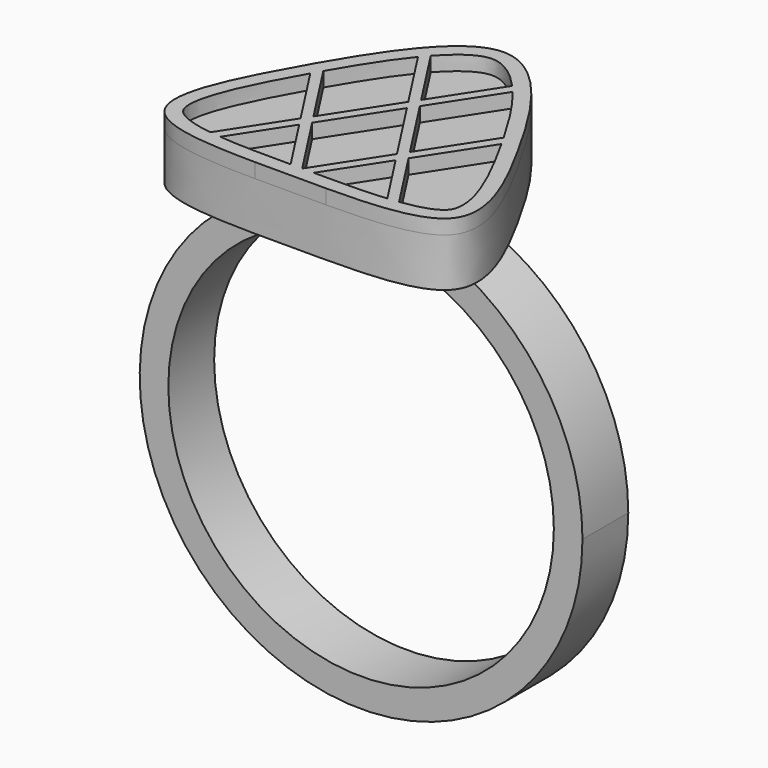
from build123d import *

# Parameters (mm, degrees)
F0_R     = 11.6
F0_R_2   = 10.1
F1_DEPTH = 3
F4_DEPTH = 2.54
F6_DEPTH = 0.762


# Not quite as in the source:
# - ends of sketch curves that miss each other by under 0.0002 mm in the source are joined
# - the dataset's text gives a spline's control points without its knots; the knots are read off the source's solid


with BuildPart() as f1:
    # F0 (on Front) → F1 (new body)
    with BuildSketch(Plane.XZ):
        Circle(F0_R)
        Circle(F0_R_2, mode=Mode.SUBTRACT)
    extrude(amount=F1_DEPTH)

    # F3 (on offset) → F4 (join)
    with BuildSketch(Plane.XY.offset(11.5951)):
        with BuildLine():
            add(Edge.make_bspline(
                [(0, 6.35), (-2.0779078975, 6.35), (-5.972334255, 0.1462705205), (-9.7622210706, -7.761600403), (0, -7.5463996638), (9.7622210706, -7.761600403), (5.972334255, 0.1462705205), (2.0779078975, 6.35), (0, 6.35)],
                knots=[0, 0, 0, 0, 0.1772793323, 0.3322578951, 0.5, 0.6677421049, 0.8227206677, 1, 1, 1, 1], degree=3))
        make_face()
    extrude(amount=F4_DEPTH)

    # F5 (on face) → F6 (join)
    with BuildSketch(Plane.XY.offset(14.1351)):
        with BuildLine():
            add(Edge.make_bspline(
                [(1.8621309249, -7.6179364202), (4.5064725103, -7.597781529), (9.5238408191, -7.2642028945), (5.972334255, 0.1462705205), (2.0779078975, 6.35), (0, 6.35)],
                knots=[0.5314495212, 0.5314495212, 0.5314495212, 0.5314495212, 0.6677421049, 0.8227206677, 1, 1, 1, 1], degree=3))
            add(Edge.make_bspline(
                [(0, 6.35), (-2.0779078975, 6.35), (-5.972334255, 0.1462705205), (-9.5238408191, -7.2642028945), (-4.5064725103, -7.597781529), (-1.8621309249, -7.6179364202)],
                knots=[0, 0, 0, 0, 0.1772793323, 0.3322578951, 0.4685504788, 0.4685504788, 0.4685504788, 0.4685504788], degree=3))
            add(Edge.make_bspline(
                [(-1.8621309249, -7.6179364202), (-1.2480712309, -7.573857345), (0, -7.5189419826), (1.2480712309, -7.573857345), (1.8621309249, -7.6179364202)],
                knots=[0.4788567979, 0.4788567979, 0.4788567979, 0.4788567979, 0.5, 0.5211432021, 0.5211432021, 0.5211432021, 0.5211432021], degree=3))
        make_face()
        with BuildLine():
            add(Edge.make_bspline(
                [(-2.4816082782, 3.8281001657), (-2.5343802796, 3.7637274985), (-2.9162768938, 3.2882987067), (-3.6254819159, 2.2796916192), (-4.3137688684, 1.1448648199), (-4.6726591189, 0.5221257557), (-4.7250085334, 0.4306953674)],
                knots=[0.088736613, 0.088736613, 0.088736613, 0.088736613, 0.09375, 0.125, 0.15625, 0.1616197523, 0.1616197523, 0.1616197523, 0.1616197523], degree=3))
            add(Edge.make_bspline(
                [(-2.1365586498, 4.2296753486), (-2.2511551272, 4.102891236), (-2.366322216, 3.9687291188), (-2.4816082782, 3.8281001657)],
                knots=[0.0777843348, 0.0777843348, 0.0777843348, 0.0777843348, 0.088736613, 0.088736613, 0.088736613, 0.088736613], degree=3))
            add(Edge.make_bspline(
                [(0, 5.588), (-0.0564230571, 5.588), (-0.1692691714, 5.580201891), (-0.4101970388, 5.5316620699), (-0.7423807218, 5.4027827261), (-1.186352477, 5.126577291), (-1.6554698528, 4.7353575108), (-1.9766347616, 4.4066075606), (-2.1365586498, 4.2296753486)],
                knots=[0, 0, 0, 0, 0.0078125, 0.015625, 0.03125, 0.046875, 0.0625, 0.0777843348, 0.0777843348, 0.0777843348, 0.0777843348], degree=3))
            add(Edge.make_bspline(
                [(2.1365586498, 4.2296753486), (1.9766347616, 4.4066075606), (1.6554698528, 4.7353575108), (1.186352477, 5.126577291), (0.7423807218, 5.4027827261), (0.4101970388, 5.5316620699), (0.1692691714, 5.580201891), (0.0564230571, 5.588), (0, 5.588)],
                knots=[0.9222156652, 0.9222156652, 0.9222156652, 0.9222156652, 0.9375, 0.953125, 0.96875, 0.984375, 0.9921875, 1, 1, 1, 1], degree=3))
            add(Edge.make_bspline(
                [(2.4816082782, 3.8281001657), (2.366322216, 3.9687291188), (2.2511551272, 4.102891236), (2.1365586498, 4.2296753486)],
                knots=[0.911263387, 0.911263387, 0.911263387, 0.911263387, 0.9222156652, 0.9222156652, 0.9222156652, 0.9222156652], degree=3))
            add(Edge.make_bspline(
                [(4.7250085334, 0.4306953674), (4.6726591189, 0.5221257557), (4.3137688684, 1.1448648199), (3.6254819159, 2.2796916192), (2.9162768938, 3.2882987067), (2.5343802796, 3.7637274985), (2.4816082782, 3.8281001657)],
                knots=[0.8383802477, 0.8383802477, 0.8383802477, 0.8383802477, 0.84375, 0.875, 0.90625, 0.911263387, 0.911263387, 0.911263387, 0.911263387], degree=3))
            add(Edge.make_bspline(
                [(5.0073229685, -0.0677201042), (4.9141625319, 0.0983598325), (4.8200413076, 0.26471675), (4.7250085334, 0.4306953674)],
                knots=[0.8286322408, 0.8286322408, 0.8286322408, 0.8286322408, 0.8383802477, 0.8383802477, 0.8383802477, 0.8383802477], degree=3))
            add(Edge.make_bspline(
                [(4.9439608161, -6.6925174845), (4.9858176889, -6.6868380172), (5.254154786, -6.6488274862), (5.7121852058, -6.5640205362), (6.2365479646, -6.4129993057), (6.6366004374, -6.2332169395), (6.8546525359, -6.0751763267), (6.9682464356, -5.9541298184), (7.0495464906, -5.8365993116), (7.1250231512, -5.653747574), (7.1675880901, -5.3285920553), (7.1372157684, -4.8940903912), (7.0250329785, -4.3683523575), (6.770198138, -3.5694722363), (6.2740558144, -2.4244183762), (5.6110952095, -1.1558825717), (5.1662615974, -0.351188467), (5.0121706035, -0.0763621301), (5.0073229685, -0.0677201042)],
                knots=[0.5909001737, 0.5909001737, 0.5909001737, 0.5909001737, 0.59375, 0.609375, 0.625, 0.640625, 0.65625, 0.6640625, 0.671875, 0.6875, 0.703125, 0.71875, 0.734375, 0.75, 0.78125, 0.8125, 0.828125, 0.8286322408, 0.8286322408, 0.8286322408, 0.8286322408], degree=3))
            add(Edge.make_bspline(
                [(4.3797296074, -6.7559609058), (4.5755658638, -6.7379434213), (4.7640552636, -6.7169284748), (4.9439608161, -6.6925174845)],
                knots=[0.5786512993, 0.5786512993, 0.5786512993, 0.5786512993, 0.5909001737, 0.5909001737, 0.5909001737, 0.5909001737], degree=3))
            add(Edge.make_bspline(
                [(0.6050961097, -6.8584772032), (0.7141147867, -6.8585902422), (1.1322874105, -6.8589569218), (2.154823412, -6.8572987447), (3.3261548926, -6.8341482776), (4.1215009809, -6.7797186631), (4.3797296074, -6.7559609058)],
                knots=[0.5101325373, 0.5101325373, 0.5101325373, 0.5101325373, 0.515625, 0.53125, 0.5625, 0.5786512993, 0.5786512993, 0.5786512993, 0.5786512993], degree=3))
            add(Edge.make_bspline(
                [(0, -6.858), (0.2019888096, -6.858), (0.4039776193, -6.8582686681), (0.6050961097, -6.8584772032)],
                knots=[0.5, 0.5, 0.5, 0.5, 0.5101325373, 0.5101325373, 0.5101325373, 0.5101325373], degree=3))
            add(Edge.make_bspline(
                [(-0.6050961097, -6.8584772032), (-0.4039776193, -6.8582686681), (-0.2019888096, -6.858), (0, -6.858)],
                knots=[0.4898674627, 0.4898674627, 0.4898674627, 0.4898674627, 0.5, 0.5, 0.5, 0.5], degree=3))
            add(Edge.make_bspline(
                [(-4.3797296074, -6.7559609058), (-4.1215009809, -6.7797186631), (-3.3261548926, -6.8341482776), (-2.154823412, -6.8572987447), (-1.1322874105, -6.8589569218), (-0.7141147867, -6.8585902422), (-0.6050961097, -6.8584772032)],
                knots=[0.4213487007, 0.4213487007, 0.4213487007, 0.4213487007, 0.4375, 0.46875, 0.484375, 0.4898674627, 0.4898674627, 0.4898674627, 0.4898674627], degree=3))
            add(Edge.make_bspline(
                [(-4.9439608161, -6.6925174845), (-4.7640552636, -6.7169284748), (-4.5755658638, -6.7379434213), (-4.3797296074, -6.7559609058)],
                knots=[0.4090998263, 0.4090998263, 0.4090998263, 0.4090998263, 0.4213487007, 0.4213487007, 0.4213487007, 0.4213487007], degree=3))
            add(Edge.make_bspline(
                [(-5.0073229685, -0.0677201042), (-5.0121706035, -0.0763621301), (-5.1662615974, -0.351188467), (-5.6110952095, -1.1558825717), (-6.2740558144, -2.4244183762), (-6.770198138, -3.5694722363), (-7.0250329785, -4.3683523575), (-7.1372157684, -4.8940903912), (-7.1675880901, -5.3285920553), (-7.1250231512, -5.653747574), (-7.0495464906, -5.8365993116), (-6.9682464356, -5.9541298184), (-6.8546525359, -6.0751763267), (-6.6366004374, -6.2332169395), (-6.2365479646, -6.4129993057), (-5.7121852058, -6.5640205362), (-5.254154786, -6.6488274862), (-4.9858176889, -6.6868380172), (-4.9439608161, -6.6925174845)],
                knots=[0.1713677592, 0.1713677592, 0.1713677592, 0.1713677592, 0.171875, 0.1875, 0.21875, 0.25, 0.265625, 0.28125, 0.296875, 0.3125, 0.328125, 0.3359375, 0.34375, 0.359375, 0.375, 0.390625, 0.40625, 0.4090998263, 0.4090998263, 0.4090998263, 0.4090998263], degree=3))
            add(Edge.make_bspline(
                [(-4.7250085334, 0.4306953674), (-4.8200413076, 0.26471675), (-4.9141625319, 0.0983598325), (-5.0073229685, -0.0677201042)],
                knots=[0.1616197523, 0.1616197523, 0.1616197523, 0.1616197523, 0.1713677592, 0.1713677592, 0.1713677592, 0.1713677592], degree=3))
        make_face(mode=Mode.SUBTRACT)
        with BuildLine():
            add(Edge.make_bspline(
                [(-1.8621309249, -7.6179364202), (-1.2480712309, -7.573857345), (0, -7.5189419826), (1.2480712309, -7.573857345), (1.8621309249, -7.6179364202)],
                knots=[0.4788567979, 0.4788567979, 0.4788567979, 0.4788567979, 0.5, 0.5211432021, 0.5211432021, 0.5211432021, 0.5211432021], degree=3))
            add(Edge.make_bspline(
                [(-1.8621309249, -7.6179364202), (-1.2519489581, -7.6225871624), (0, -7.6174128376), (1.2519489581, -7.6225871624), (1.8621309249, -7.6179364202)],
                knots=[0.4685504788, 0.4685504788, 0.4685504788, 0.4685504788, 0.5, 0.5314495212, 0.5314495212, 0.5314495212, 0.5314495212], degree=3))
        make_face()
        with BuildLine():
            add(Edge.make_bspline(
                [(-2.1365586498, 4.2296753486), (-2.2511551272, 4.102891236), (-2.366322216, 3.9687291188), (-2.4816082782, 3.8281001657)],
                knots=[0.0777843348, 0.0777843348, 0.0777843348, 0.0777843348, 0.088736613, 0.088736613, 0.088736613, 0.088736613], degree=3))
            Line((-2.4816082782, 3.8281001657), (-0.3027027565, 0.4669405984))
            Line((-0.3027027565, 0.4669405984), (-2.525614526, -2.9620594016))
            Line((-2.525614526, -2.9620594016), (-4.7250421363, 0.4307146071))
            add(Edge.make_bspline(
                [(-4.7250421363, 0.4307146071), (-4.8200413076, 0.26471675), (-4.9141625319, 0.0983598325), (-5.0073229685, -0.0677201042)],
                knots=[0.1616197523, 0.1616197523, 0.1616197523, 0.1616197523, 0.1713677592, 0.1713677592, 0.1713677592, 0.1713677592], degree=3))
            Line((-5.0073229685, -0.0677201042), (-2.8283172825, -3.429))
            Line((-2.8283172825, -3.429), (-4.9439631514, -6.6925346952))
            add(Edge.make_bspline(
                [(-4.9439631514, -6.6925346952), (-4.7640552636, -6.7169284748), (-4.5755658638, -6.7379434213), (-4.3797296074, -6.7559609058)],
                knots=[0.4090998263, 0.4090998263, 0.4090998263, 0.4090998263, 0.4213487007, 0.4213487007, 0.4213487007, 0.4213487007], degree=3))
            Line((-4.3797296074, -6.7559609058), (-2.525614526, -3.8959405984))
            Line((-2.525614526, -3.8959405984), (-0.6050961096, -6.8584772767))
            add(Edge.make_bspline(
                [(-0.6050961096, -6.8584772767), (-0.4039776193, -6.8582686681), (-0.2019888096, -6.858), (0, -6.858)],
                knots=[0.4898674627, 0.4898674627, 0.4898674627, 0.4898674627, 0.5, 0.5, 0.5, 0.5], degree=3))
            add(Edge.make_bspline(
                [(0, -6.858), (0.2019888096, -6.858), (0.4039776193, -6.8582686681), (0.6050961097, -6.8584772032)],
                knots=[0.5, 0.5, 0.5, 0.5, 0.5101325373, 0.5101325373, 0.5101325373, 0.5101325373], degree=3))
            Line((0.6050961097, -6.8584772032), (2.525614526, -3.8959405984))
            Line((2.525614526, -3.8959405984), (4.3797386663, -6.7560593687))
            add(Edge.make_bspline(
                [(4.3797386663, -6.7560593687), (4.5755658638, -6.7379434213), (4.7640552636, -6.7169284748), (4.9439608161, -6.6925174845)],
                knots=[0.5786512993, 0.5786512993, 0.5786512993, 0.5786512993, 0.5909001737, 0.5909001737, 0.5909001737, 0.5909001737], degree=3))
            Line((4.9439608161, -6.6925174845), (2.8283172825, -3.429))
            Line((2.8283172825, -3.429), (5.0073312834, -0.0677154401))
            add(Edge.make_bspline(
                [(5.0073312834, -0.0677154401), (4.9141625319, 0.0983598325), (4.8200413076, 0.26471675), (4.7250085334, 0.4306953674)],
                knots=[0.8286322408, 0.8286322408, 0.8286322408, 0.8286322408, 0.8383802477, 0.8383802477, 0.8383802477, 0.8383802477], degree=3))
            Line((4.7250085334, 0.4306953674), (2.525614526, -2.9620594016))
            Line((2.525614526, -2.9620594016), (0.3027027565, 0.4669405984))
            Line((0.3027027565, 0.4669405984), (2.4816668633, 3.8281481931))
            add(Edge.make_bspline(
                [(2.4816668633, 3.8281481931), (2.366322216, 3.9687291188), (2.2511551272, 4.102891236), (2.1365586498, 4.2296753486)],
                knots=[0.911263387, 0.911263387, 0.911263387, 0.911263387, 0.9222156652, 0.9222156652, 0.9222156652, 0.9222156652], degree=3))
            Line((2.1365586498, 4.2296753486), (0, 0.9338811968))
            Line((0, 0.9338811968), (-2.1365586498, 4.2296753486))
        make_face()
        Polygon((2.2229117696, -3.429), (0, -6.858), (-2.2229117696, -3.429), (0, 0), align=None, mode=Mode.SUBTRACT)
    extrude(amount=F6_DEPTH)


solid = f1.part
